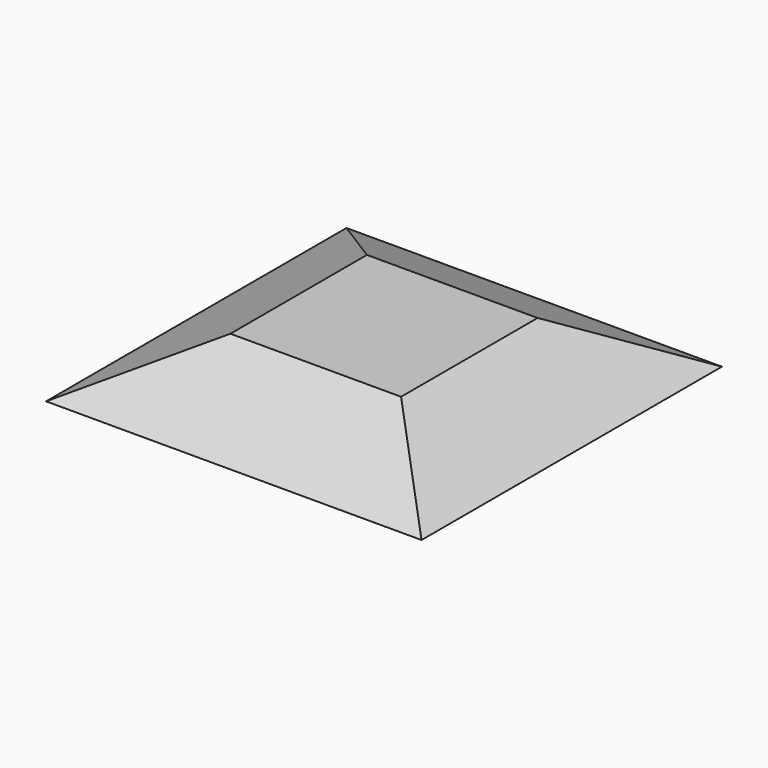
from build123d import *

# Parameters (mm, degrees)
F0_W       = 63.5
F0_H       = 38.1
F1_DEPTH   = 279.4
F2_SIZE2   = 76.19999
F2_SIZE    = 38.09999
F2_2_SIZE2 = 76.19999
F2_2_SIZE  = 38.09999


# Not quite as in the source:
# - a fillet or chamfer is up to 0.001 mm smaller than in the source, because OpenCascade refuses the exact size


with BuildPart() as f1:
    # F0 (on Front) → F1 (new body)
    with BuildSketch(Plane.XZ):
        with Locations((-31.75, -19.05)):
            Rectangle(F0_W, F0_H)
        Polygon((0, 0), (0, -38.1), (139.7, -38.1), (63.5, 0), align=None)
        Polygon((-63.5, 0), (-139.7, -38.1), (-63.5, -38.1), align=None)
    extrude(amount=F1_DEPTH)

    # F2 (size 38.1 and 76.2 in the source; OpenCascade refuses exactly that, so slightly less here)
    f2_edges = [f1.edges().sort_by_distance(p)[0] for p in [
        (0, -279.4, 0),
    ]]
    f2_side = f1.faces().sort_by_distance((0, -279.4, -21.43125))[0]
    chamfer(f2_edges, length=F2_SIZE, length2=F2_SIZE2, reference=f2_side)

    # F2#2 (size 38.1 and 76.2 in the source; OpenCascade refuses exactly that, so slightly less here)
    f2_2_edges = [f1.edges().sort_by_distance(p)[0] for p in [
        (0, 0, 0),
    ]]
    f2_2_side = f1.faces().sort_by_distance((0, 0, -21.43125))[0]
    chamfer(f2_2_edges, length=F2_2_SIZE, length2=F2_2_SIZE2, reference=f2_2_side)


solid = f1.part
